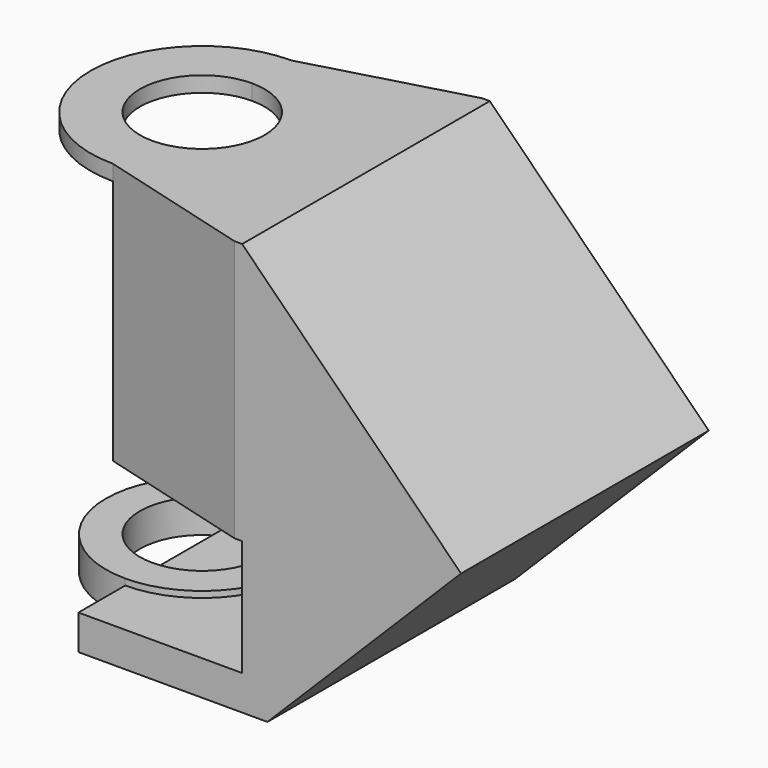
from build123d import *

# Parameters (mm, degrees)
F1_DEPTH = 31.8
F2_DEPTH = 31.8
F3_DEPTH = 2
F4_DEPTH = 1
F6_START = -46
F6_DEPTH = 4.3
F7_DEPTH = 40


with BuildPart() as f1:
    # F0 (on Top) → F1 (new body)
    with BuildSketch(Plane.XY):
        with BuildLine():
            ThreePointArc((0, 12.44), (8.796408358, 8.796408358), (12.44, 0))
            ThreePointArc((12.44, 0), (8.796408358, -8.796408358), (0, -12.44))
            Line((0, -12.44), (0, -14.44))
            ThreePointArc((0, -14.44), (10.2106219203, -10.2106219203), (14.44, 0))
            ThreePointArc((14.44, 0), (10.2106219203, 10.2106219203), (0, 14.44))
            Line((0, 14.44), (0, 12.44))
        make_face()
    extrude(amount=-F1_DEPTH)

    # F0 (on Top) → F2 (join)
    with BuildSketch(Plane.XY):
        with BuildLine():
            add(Edge.make_bspline(
                [(0, 14.44), (6.7187255869, 16.2933333333), (13.4374511739, 18.1466666667), (20.1561767608, 20)],
                knots=[0, 0, 0, 0, 20.9089708406, 20.9089708406, 20.9089708406, 20.9089708406], degree=3))
            ThreePointArc((0, 14.44), (10.2106219203, 10.2106219203), (14.44, 0))
            ThreePointArc((14.44, 0), (10.2106219203, -10.2106219203), (0, -14.44))
            add(Edge.make_bspline(
                [(0, -14.44), (6.7187255869, -16.2933333333), (13.4374511739, -18.1466666667), (20.1561767608, -20)],
                knots=[0, 0, 0, 0, 20.9089708406, 20.9089708406, 20.9089708406, 20.9089708406], degree=3))
            Line((20.1561767608, -20), (20.1561767608, 20))
        make_face()
    extrude(amount=-F2_DEPTH)

    # F0 (on Top) → F3 (join)
    with BuildSketch(Plane.XY):
        with BuildLine():
            ThreePointArc((0, 12.44), (8.796408358, 8.796408358), (12.44, 0))
            ThreePointArc((12.44, 0), (8.796408358, -8.796408358), (0, -12.44))
            Line((0, -12.44), (0, -14.44))
            ThreePointArc((0, -14.44), (10.2106219203, -10.2106219203), (14.44, 0))
            ThreePointArc((14.44, 0), (10.2106219203, 10.2106219203), (0, 14.44))
            Line((0, 14.44), (0, 12.44))
        make_face()
        with BuildLine():
            ThreePointArc((0, -12.44), (8.796408358, -8.796408358), (12.44, 0))
            ThreePointArc((12.44, 0), (8.796408358, 8.796408358), (0, 12.44))
            Line((0, 12.44), (0, 8.05))
            ThreePointArc((0, 8.05), (5.6922095886, 5.6922095886), (8.05, 0))
            ThreePointArc((8.05, 0), (5.6922095886, -5.6922095886), (0, -8.05))
            Line((0, -8.05), (0, -12.44))
        make_face()
        with BuildLine():
            Line((0, 8.05), (0, 12.44))
            ThreePointArc((0, 12.44), (-12.44, 0), (0, -12.44))
            Line((0, -12.44), (0, -8.05))
            ThreePointArc((0, -8.05), (-8.05, 0), (0, 8.05))
        make_face()
        with BuildLine():
            ThreePointArc((0, -12.44), (-12.44, 0), (0, 12.44))
            Line((0, 12.44), (0, 14.44))
            ThreePointArc((0, 14.44), (-14.44, 0), (0, -14.44))
            Line((0, -14.44), (0, -12.44))
        make_face()
        with BuildLine():
            add(Edge.make_bspline(
                [(0, 14.44), (6.7187255869, 16.2933333333), (13.4374511739, 18.1466666667), (20.1561767608, 20)],
                knots=[0, 0, 0, 0, 20.9089708406, 20.9089708406, 20.9089708406, 20.9089708406], degree=3))
            ThreePointArc((0, 14.44), (10.2106219203, 10.2106219203), (14.44, 0))
            ThreePointArc((14.44, 0), (10.2106219203, -10.2106219203), (0, -14.44))
            add(Edge.make_bspline(
                [(0, -14.44), (6.7187255869, -16.2933333333), (13.4374511739, -18.1466666667), (20.1561767608, -20)],
                knots=[0, 0, 0, 0, 20.9089708406, 20.9089708406, 20.9089708406, 20.9089708406], degree=3))
            Line((20.1561767608, -20), (20.1561767608, 20))
        make_face()
    extrude(amount=F3_DEPTH)

    # F4 (add): a face of the model
    f4_faces = [f1.faces().sort_by_distance(p)[0] for p in [
        (20.1561767608, 0, -14.9),
    ]]
    extrude(f4_faces, amount=F4_DEPTH)

    # F5 (on face) → F7 (join, through all)
    with BuildSketch(Plane.XZ.offset(20)):
        Polygon((49.4404480083, -26.2842712475), (21.1561767608, 2), (21.1561767608, -31.8), (21.1561767608, -46.8), (0, -46.8), (0, -51.3), (24.4247192557, -51.3), align=None)
    extrude(amount=-F7_DEPTH)


with BuildPart() as f6:
    # F0 (on Top) → F6 (new body)
    with BuildSketch(Plane.XY.offset(F6_START)):
        with BuildLine():
            ThreePointArc((0, -12.44), (8.796408358, -8.796408358), (12.44, 0))
            ThreePointArc((12.44, 0), (8.796408358, 8.796408358), (0, 12.44))
            Line((0, 12.44), (0, 8.05))
            ThreePointArc((0, 8.05), (5.6922095886, 5.6922095886), (8.05, 0))
            ThreePointArc((8.05, 0), (5.6922095886, -5.6922095886), (0, -8.05))
            Line((0, -8.05), (0, -12.44))
        make_face()
        with BuildLine():
            Line((0, 8.05), (0, 12.44))
            ThreePointArc((0, 12.44), (-12.44, 0), (0, -12.44))
            Line((0, -12.44), (0, -8.05))
            ThreePointArc((0, -8.05), (-8.05, 0), (0, 8.05))
        make_face()
    extrude(amount=-F6_DEPTH)


solid = Compound([f1.part, f6.part])
